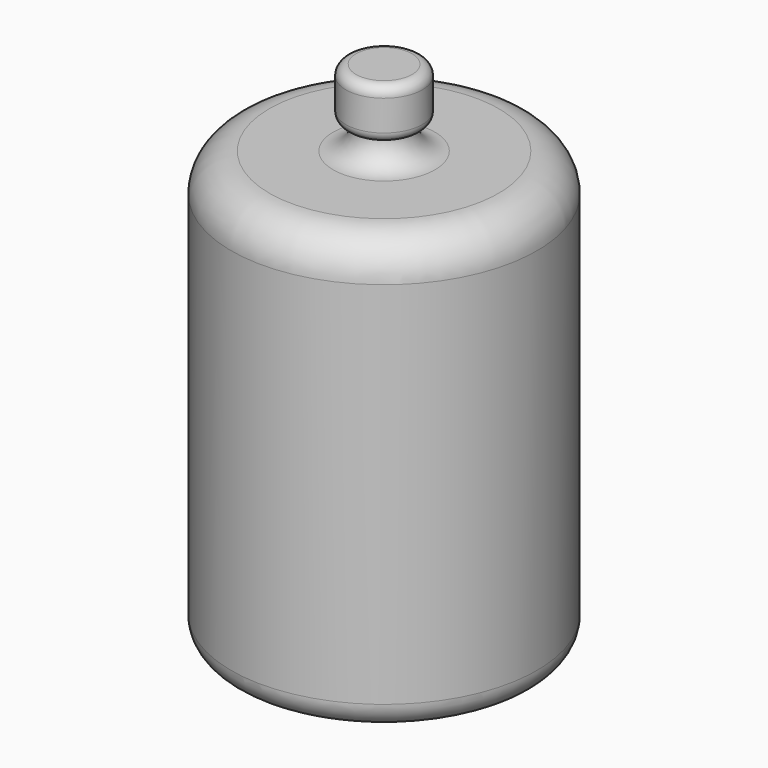
from build123d import *

# Parameters (mm, degrees)
F0_W = 76.2
F0_H = 12.7
F2_R = 19.05
F3_R = 12.7
F4_R = 12.69999
F5_R = 5.08
F6_R = 5.08


# Not quite as in the source:
# - a fillet or chamfer is up to 0.001 mm smaller than in the source, because OpenCascade refuses the exact size


with BuildPart() as f1:
    # F0 (on Front) → F1 (revolve)
    with BuildSketch(Plane.XZ):
        with Locations((-38.1, -180.2761299372)):
            Rectangle(F0_W, F0_H)
        Polygon((-76.2, -173.9261299372), (0, -173.9261299372), (0, 29.2738700628), (-12.7, 29.2738700628), (-76.2, 29.2738700628), align=None)
        Polygon((-12.7, 29.2738700628), (0, 29.2738700628), (0, 35.6238700628), (0, 41.9738700628), (-12.7, 41.9738700628), align=None)
        Polygon((-19.05, 41.9738700628), (-12.7, 41.9738700628), (0, 41.9738700628), (0, 61.0238700628), (0, 67.3738700628), (-19.05, 67.3738700628), align=None)
    revolve(axis=Axis((0, 0, -14.5017058273), (0, 0, -1)))

    # F2
    f2_edges = [f1.edges().sort_by_distance(p)[0] for p in [
        (76.2, 0, 29.27387),
    ]]
    fillet(f2_edges, radius=F2_R)

    # F3
    f3_edges = [f1.edges().sort_by_distance(p)[0] for p in [
        (76.2, 0, -186.62613),
    ]]
    fillet(f3_edges, radius=F3_R)

    # F4 (radius 12.7 in the source; OpenCascade refuses exactly that, so slightly less here)
    f4_edges = [f1.edges().sort_by_distance(p)[0] for p in [
        (12.7, 0, 29.27387),
    ]]
    fillet(f4_edges, radius=F4_R)

    # F5
    f5_edges = [f1.edges().sort_by_distance(p)[0] for p in [
        (19.05, 0, 41.97387),
    ]]
    fillet(f5_edges, radius=F5_R)

    # F6
    f6_edges = [f1.edges().sort_by_distance(p)[0] for p in [
        (19.05, 0, 67.37387),
    ]]
    fillet(f6_edges, radius=F6_R)


solid = f1.part
